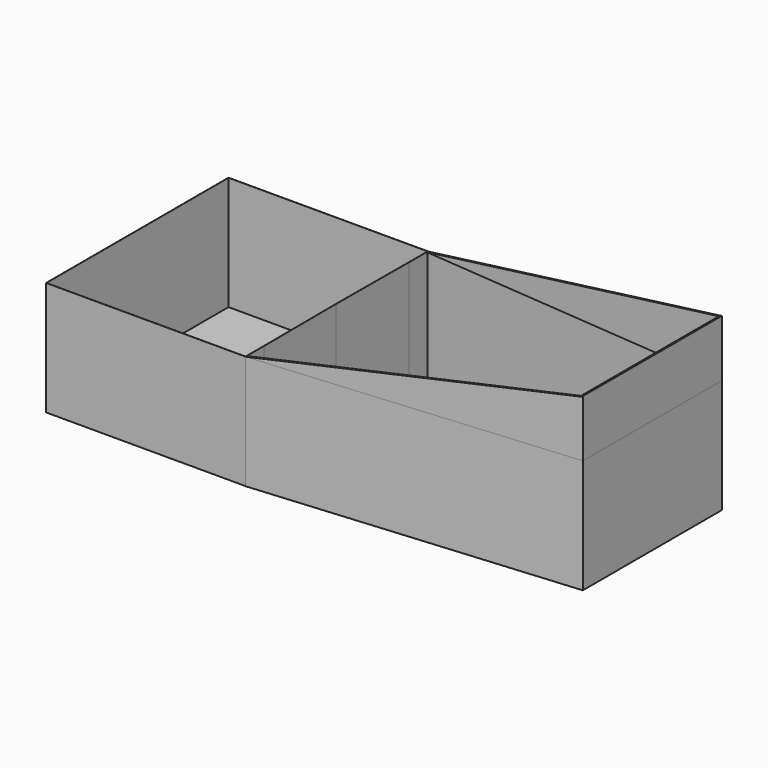
from build123d import *

# Parameters (mm, degrees)
F1_W      = 700
F1_H      = 800
F2_DEPTH  = 400
F3_T      = -0.5
F4_DEPTH  = 400
F5_T      = -0.5
F8_DEPTH  = 5
F6_W      = 610
F6_H      = 200
F9_DEPTH  = 5
F11_DEPTH = 5


# Not quite as in the source:
# - a shell that OpenCascade refuses in one call is made with other operations: the cavity is built on its own and cut out


with BuildPart() as f2:
    # F1 (on Top) → F2 (new body)
    with BuildSketch(Plane.XY):
        with Locations((-437.323653698, 0.5818843842)):
            Rectangle(F1_W, F1_H)
    extrude(amount=F2_DEPTH)

    # F3
    f3_openings = [f2.faces().sort_by_distance(p)[0] for p in [
        (-437.323654, 0.581884, 400),
    ]]
    offset(amount=F3_T, openings=f3_openings)

    # F0 (on Top) → F4 (join)
    with BuildSketch(Plane.XY):
        Polygon((-87.3838496962, 399.99429066), (-89.5210065554, 0), (1020.4789934446, 0), (1020.4789934446, 305), align=None)
        Polygon((-89.5210065554, 0), (-87.3838496962, -399.99429066), (1020.4789934446, -305), (1020.4789934446, 0), align=None)
    extrude(amount=F4_DEPTH)

    # F5: a shell. OpenCascade refuses it in one call, so the cavity is built on its own and cut out:
    # the body offset inwards by the wall thickness, plus a prism from it out through each open face.
    f5_core = offset(f2.part, amount=F5_T, kind=Kind.INTERSECTION, mode=Mode.PRIVATE)
    f5_exits = [f5_core.faces().sort_by_distance(p)[0] for p in [
        (441.073229, 0.000123, 399.5),
    ]]
    add(f5_core, mode=Mode.SUBTRACT)
    extrude(f5_exits, amount=-F5_T, mode=Mode.SUBTRACT)


with BuildPart() as f8:
    # F7 (on face) → F8 (new body)
    with BuildSketch(Plane(origin=(33.409614528, -389.6367906126, 0), x_dir=(0.9963439994, 0.0854320479, 0), z_dir=(0.0854320479, -0.9963439994, 0))):
        Polygon((990.954875946, 597.5561738014), (-121.2367056898, 400), (990.6913470501, 400), align=None)
    extrude(amount=-F8_DEPTH)


with BuildPart() as f9:
    # F6 (on face) → F9 (new body)
    with BuildSketch(Plane.YZ.offset(1020.4789934446)):
        with Locations((0, 500)):
            Rectangle(F6_W, F6_H)
    extrude(amount=-F9_DEPTH)


with BuildPart() as f11:
    # F10 (on face) → F11 (new body)
    with BuildSketch(Plane(origin=(33.409614528, 389.6367906126, 0), x_dir=(-0.9963439994, 0.0854320479, 0), z_dir=(0.0854320479, 0.9963439994, 0))):
        Polygon((121.1762888074, 400), (-990.6913470501, 599.4713306427), (-990.6913470501, 400), align=None)
    extrude(amount=-F11_DEPTH)


solid = Compound([f2.part, f8.part, f9.part, f11.part])
